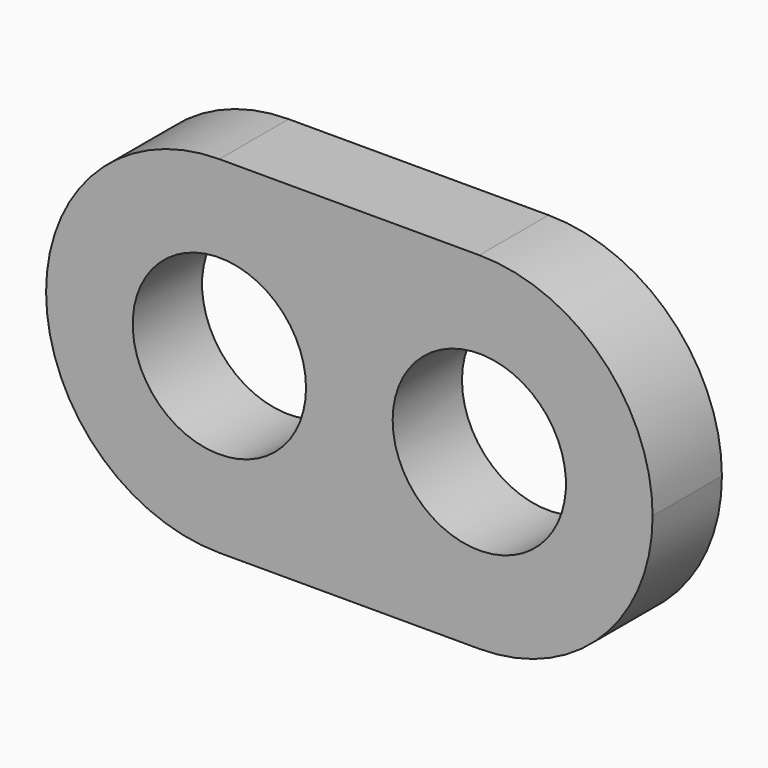
from build123d import *

# Parameters (mm, degrees)
F1_DEPTH = 25.4
F2_R     = 50.79999
F3_R     = 25.4
F4_DEPTH = 25.4


# Not quite as in the source:
# - a fillet or chamfer is up to 0.001 mm smaller than in the source, because OpenCascade refuses the exact size


with BuildPart() as f1:
    # F0 (on Front) → F1 (new body)
    with BuildSketch(Plane.XZ):
        with BuildLine():
            ThreePointArc((0, -50.8), (35.9210244843, -35.9210244843), (50.8, 0))
            ThreePointArc((50.8, 0), (35.9210244843, 35.9210244843), (0, 50.8))
            Line((0, 50.8), (0, -50.8))
        make_face()
        with BuildLine():
            ThreePointArc((0, 50.8), (35.9210244843, 35.9210244843), (50.8, 0))
            ThreePointArc((50.8, 0), (35.9210244843, -35.9210244843), (0, -50.8))
            Line((0, -50.8), (127, -50.8))
            Line((127, -50.8), (127, 50.8))
            Line((127, 50.8), (0, 50.8))
        make_face()
        with BuildLine():
            Line((0, -50.8), (0, 50.8))
            ThreePointArc((0, 50.8), (-50.8, 0), (0, -50.8))
        make_face()
    extrude(amount=F1_DEPTH)

    # F2 (radius 50.8 in the source; OpenCascade refuses exactly that, so slightly less here)
    f2_edges = [f1.edges().sort_by_distance(p)[0] for p in [
        (127, -12.7, 50.8),
        (127, -12.7, -50.8),
    ]]
    fillet(f2_edges, radius=F2_R)

    # F3 (on Front) → F4 (cut)
    with BuildSketch(Plane.XZ):
        Circle(F3_R)
    f4 = extrude(amount=F4_DEPTH, mode=Mode.SUBTRACT)

    # F6: F4 across plane
    add(f4.mirror(Plane.YZ.offset(38.1)), mode=Mode.SUBTRACT)


solid = f1.part
